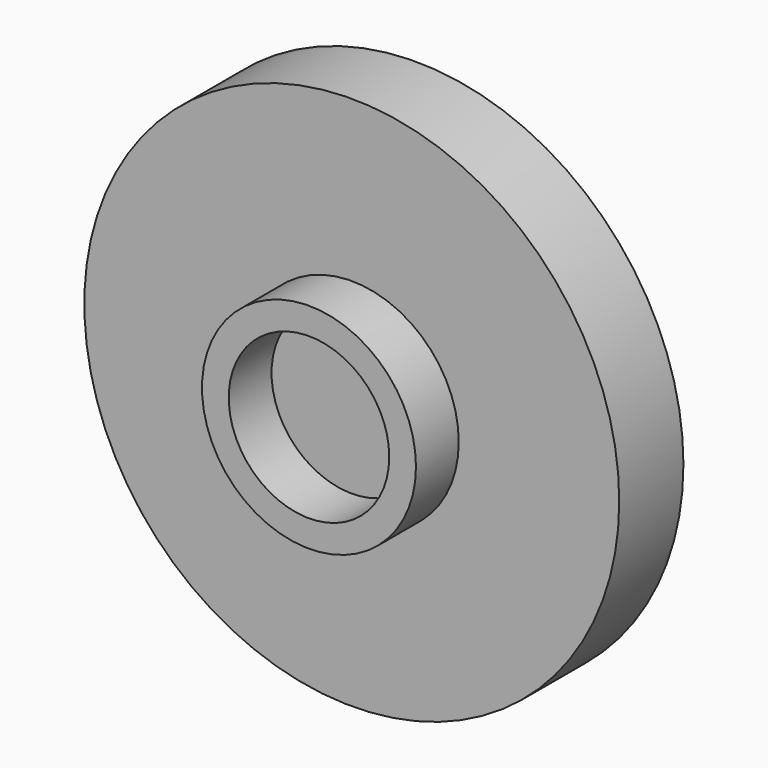
from build123d import *

# Parameters (mm, degrees)
F0_R     = 50
F1_DEPTH = 15
F3_R     = 20
F4_DEPTH = 25
F2_R     = 15


with BuildPart() as f1:
    # F0 (on Front) → F1 (new body)
    with BuildSketch(Plane.XZ):
        Circle(F0_R)
    extrude(amount=F1_DEPTH)


with BuildPart() as f4:
    # F3 (on Front) → F4 (new body)
    with BuildSketch(Plane.XZ):
        Circle(F3_R)
    extrude(amount=F4_DEPTH)


with BuildPart() as f4b:
    # F2 (on Front) → F4, piece 2 (new body)
    with BuildSketch(Plane.XZ):
        Circle(F2_R)
    extrude(amount=F4_DEPTH)


with BuildPart() as f4_1:
    add(f4.part)

    # F5: cut F4b
    add(f4b.part, mode=Mode.SUBTRACT)


solid = Compound([f1.part, f4_1.part])
